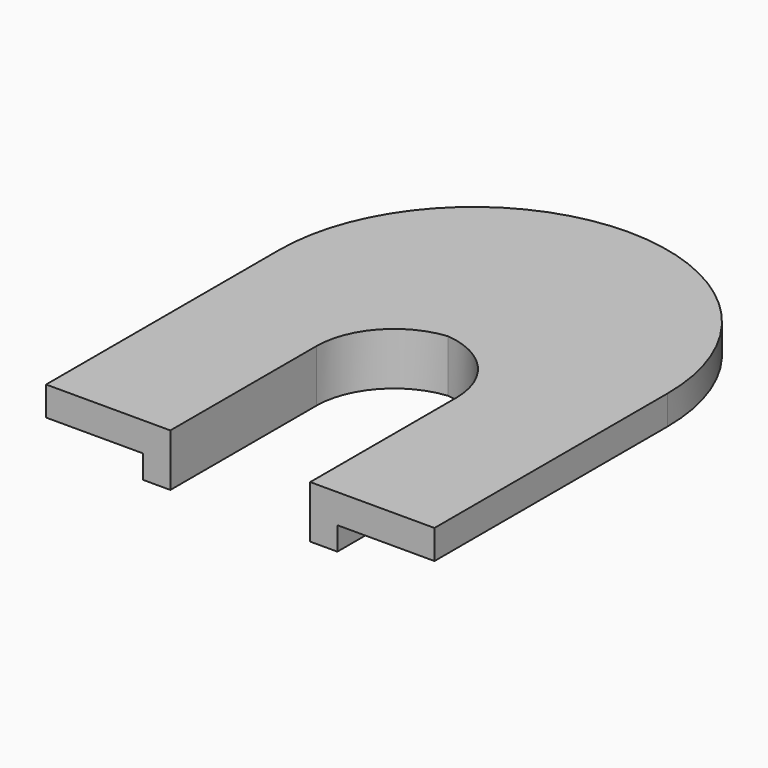
from build123d import *

# Parameters (mm, degrees)
F1_DEPTH    = 2.7
F2_T1_DEPTH = 2.7
F3_R        = 9.99999
F5_DEPTH    = 1.2


# Not quite as in the source:
# - a fillet or chamfer that OpenCascade refuses, or shapes differently, is made with other operations: its cross-section is extruded or revolved along the edge and cut away or added
# - a fillet or chamfer is up to 0.001 mm smaller than in the source, because OpenCascade refuses the exact size


with BuildPart() as f1:
    # F0 (on Top) → F1 (new body)
    with BuildSketch(Plane.XY):
        Polygon((-10, 0), (-3.6, 0), (-3.6, 13.4), (0, 13.4), (3.6, 13.4), (3.6, 0), (10, 0), (10, 25), (0, 25), (-10, 25), align=None)
    extrude(amount=F1_DEPTH)

    # F2: fillet of radius 4 on 2 edges, made by hand

    # F2_s2 → F2_t1 (join)
    with BuildSketch(Plane.XY):
        with BuildLine():
            ThreePointArc((0.4, 13.4), (-2.4284271247, 12.2284271247), (-3.6, 9.4))
            Line((-3.6, 9.4), (-3.6, 13.4))
            Line((-3.6, 13.4), (0.4, 13.4))
        make_face()
        with BuildLine():
            ThreePointArc((3.6, 9.4), (2.4284271247, 12.2284271247), (-0.4, 13.4))
            Line((-0.4, 13.4), (3.6, 13.4))
            Line((3.6, 13.4), (3.6, 9.4))
        make_face()
    extrude(amount=F2_T1_DEPTH)

    # F3 (radius 10 in the source; OpenCascade refuses exactly that, so slightly less here)
    f3_edges = [f1.edges().sort_by_distance(p)[0] for p in [
        (-10, 25, 1.35),
        (10, 25, 1.35),
    ]]
    fillet(f3_edges, radius=F3_R)

    # F4 (on Top) → F5 (cut)
    with BuildSketch(Plane.XY):
        with BuildLine():
            Line((-11.2521313131, -1.0476741055), (-5, -1.0476741055))
            Line((-5, -1.0476741055), (-5, 10))
            ThreePointArc((-5, 10), (-3.5355339059, 13.5355339059), (0, 15))
            ThreePointArc((0, 15), (3.5355339059, 13.5355339059), (5, 10))
            Line((5, 10), (5, -1.0476741055))
            Line((5, -1.0476741055), (11.2521313131, -1.0476741055))
            Line((11.2521313131, -1.0476741055), (11.2521313131, 27.1253902465))
            Line((11.2521313131, 27.1253902465), (0, 27.1253902465))
            Line((0, 27.1253902465), (-11.2521313131, 27.1253902465))
            Line((-11.2521313131, 27.1253902465), (-11.2521313131, -1.0476741055))
        make_face()
    extrude(amount=F5_DEPTH, mode=Mode.SUBTRACT)


solid = f1.part
